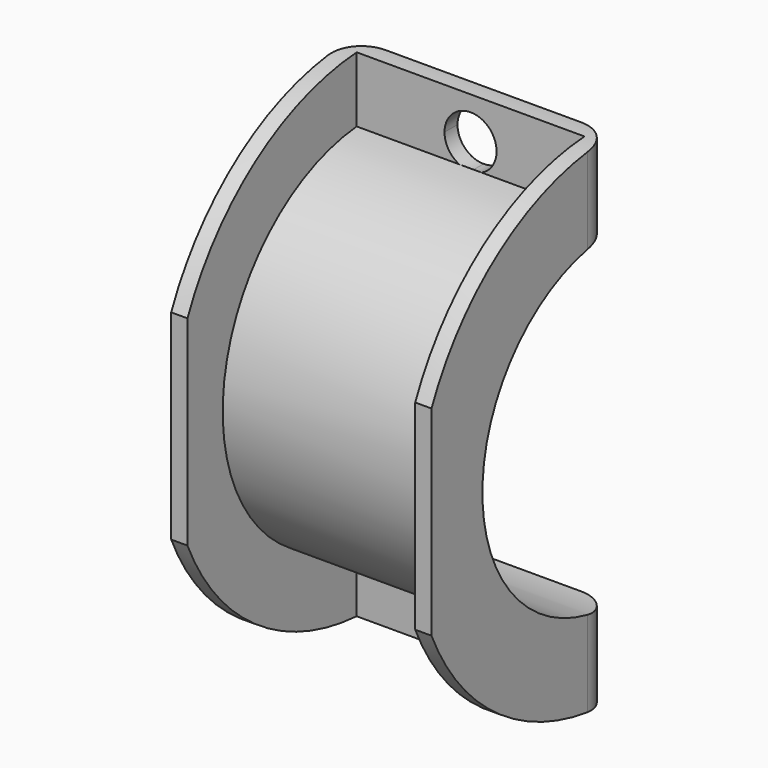
from build123d import *

# Parameters (mm, degrees)
F0_W      = 40
F0_H      = 40
F0_W_2    = 35
F0_H_2    = 35
F1_DEPTH  = 100
F3_DEPTH  = 40.001
F4_DEPTH  = 40
F5_R      = 5
F6_DEPTH  = 40
F7_R      = 5
F9_DEPTH  = 2.5
F11_DEPTH = 2.5


# Not quite as in the source:
# - a feature names something its author has since deleted; it is built from what else it names


with BuildPart() as f1:
    # F0 (on Top) → F1 (new body)
    with BuildSketch(Plane.XY):
        Rectangle(F0_W, F0_H)
        Rectangle(F0_W_2, F0_H_2, mode=Mode.SUBTRACT)
    extrude(amount=F1_DEPTH)

    # F2 (on face) → F3 (cut, through all)
    with BuildSketch(Plane.YZ.offset(20)):
        with BuildLine():
            Line((20, 25.3402171373), (20, 75.7902171373))
            ThreePointArc((20, 75.7902171373), (-5.225, 50.5652171373), (20, 25.3402171373))
        make_face()
        with BuildLine():
            ThreePointArc((20, 25.3402171373), (-5.225, 50.5652171373), (20, 75.7902171373))
            Line((20, 75.7902171373), (20, 78.7902171373))
            ThreePointArc((20, 78.7902171373), (-8.225, 50.5652171373), (20, 22.3402171373))
            Line((20, 22.3402171373), (20, 25.3402171373))
        make_face()
    extrude(amount=-F3_DEPTH, mode=Mode.SUBTRACT)

    # F2 (on face) → F4 (join)
    with BuildSketch(Plane.YZ.offset(20)):
        with BuildLine():
            ThreePointArc((20, 25.3402171373), (-5.225, 50.5652171373), (20, 75.7902171373))
            Line((20, 75.7902171373), (20, 78.7902171373))
            ThreePointArc((20, 78.7902171373), (-8.225, 50.5652171373), (20, 22.3402171373))
            Line((20, 22.3402171373), (20, 25.3402171373))
        make_face()
    extrude(amount=-F4_DEPTH)

    # F5
    f5_edges = [f1.edges().sort_by_distance(p)[0] for p in [
        (-20, -20, 50),
        (20, -20, 50),
    ]]
    fillet(f5_edges, radius=F5_R)

    # F2 (on face) → F6 (cut)
    with BuildSketch(Plane.YZ.offset(20)):
        with BuildLine():
            ThreePointArc((-15, 65.9324102773), (-0.9014313771, 82.569604202), (20, 88.7902171373))
            Line((20, 88.7902171373), (20, 100))
            Line((20, 100), (-20, 100))
            Line((-20, 100), (-20, 70.5652171373))
            Line((-20, 70.5652171373), (-20, 30.5652171373))
            Line((-20, 30.5652171373), (-20, 0))
            Line((-20, 0), (20, 0))
            Line((20, 0), (20, 12.3402171373))
            ThreePointArc((20, 12.3402171373), (-0.9014313771, 18.5608300726), (-15, 35.1980239974))
            Line((-15, 35.1980239974), (-15, 65.9324102773))
        make_face()
    extrude(amount=-F6_DEPTH, mode=Mode.SUBTRACT)

    # F7
    f7_edges = [f1.edges().sort_by_distance(p)[0] for p in [
        (-20, 20, 82.290217),
        (20, 20, 82.290217),
        (-20, 20, 18.840217),
        (20, 20, 18.840217),
    ]]
    fillet(f7_edges, radius=F7_R)

    # F8 (on face) → F9 (cut)
    with BuildSketch(Plane(origin=(0, 20, 0), x_dir=(-1, 0, 0), z_dir=(0, 1, 0))):
        with BuildLine():
            ThreePointArc((0, 86.2902171373), (-4, 82.2902171373), (0, 78.2902171373))
            Line((0, 78.2902171373), (0, 86.2902171373))
        make_face()
        with BuildLine():
            Line((0, 86.2902171373), (0, 78.2902171373))
            ThreePointArc((0, 78.2902171373), (2.8284271247, 79.4617900126), (4, 82.2902171373))
            ThreePointArc((4, 82.2902171373), (2.8284271247, 85.1186442621), (0, 86.2902171373))
        make_face()
    extrude(amount=-F9_DEPTH, mode=Mode.SUBTRACT)

    # F10 (on face) → F11 (cut)
    with BuildSketch(Plane(origin=(0, 20, 0), x_dir=(-1, 0, 0), z_dir=(0, 1, 0))):
        with BuildLine():
            ThreePointArc((0, 22.8402171373), (-4, 18.8402171373), (0, 14.8402171373))
            Line((0, 14.8402171373), (0, 22.8402171373))
        make_face()
        with BuildLine():
            Line((0, 22.8402171373), (0, 14.8402171373))
            ThreePointArc((0, 14.8402171373), (2.8284271247, 16.0117900126), (4, 18.8402171373))
            ThreePointArc((4, 18.8402171373), (2.8284271247, 21.6686442621), (0, 22.8402171373))
        make_face()
    extrude(amount=-F11_DEPTH, mode=Mode.SUBTRACT)


solid = f1.part
